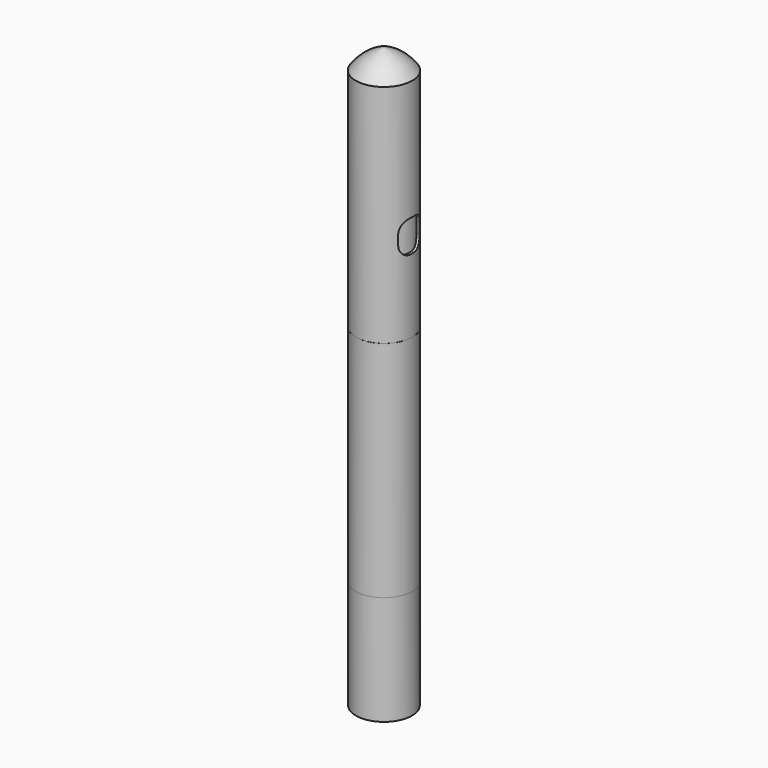
from build123d import *

# Parameters (mm, degrees)
F2_T     = -1
F4_DEPTH = 21.9
F6_E12_W = 45.703087002
F6_E12_H = 50
F7_DEPTH = 0.01


with BuildPart() as f1:
    # F0 (on Front) → F1 (revolve)
    with BuildSketch(Plane.XZ):
        with BuildLine():
            Line((-10.5, -33.0094280231), (0, -33.0094280231))
            Line((0, -33.0094280231), (0, 176.4999798387))
            Line((0, 176.4999798387), (0, 183.9905719769))
            ThreePointArc((0, 183.9905719769), (-5.9594664964, 181.1784924991), (-10.6, 176.4999798387))
            Line((-10.6, 176.4999798387), (-10.6, 7.9905719769))
            Line((-10.6, 7.9905719769), (-10.5, 7.9905719769))
            Line((-10.5, 7.9905719769), (-10.5, -33.0094280231))
        make_face()
    revolve(axis=Axis((0, 0, 180.2452759078), (0, 0, 1)))

    # F2
    f2_openings = [f1.faces().sort_by_distance(p)[0] for p in [
        (0, 0, -33.009428),
    ]]
    offset(amount=F2_T, openings=f2_openings, kind=Kind.INTERSECTION)

    # F3 (on Right) → F4 (cut)
    with BuildSketch(Plane.YZ):
        with BuildLine():
            ThreePointArc((5, 127.4999798387), (3.8284271247, 130.3284069635), (1, 131.4999798387))
            Line((1, 131.4999798387), (-1, 131.4999798387))
            ThreePointArc((-1, 131.4999798387), (-3.8284271247, 130.3284069635), (-5, 127.4999798387))
            Line((-5, 127.4999798387), (-5, 123.4999798387))
            ThreePointArc((-5, 123.4999798387), (-3.8284271247, 120.671552714), (-1, 119.4999798387))
            Line((-1, 119.4999798387), (1, 119.4999798387))
            ThreePointArc((1, 119.4999798387), (3.8284271247, 120.671552714), (5, 123.4999798387))
            Line((5, 123.4999798387), (5, 127.4999798387))
        make_face()
    extrude(amount=F4_DEPTH, mode=Mode.SUBTRACT)

    # F6_E12 (on explicit) → F7 (cut)
    with BuildSketch(Plane(origin=(-25, 19.7467152029, 91.902948916), x_dir=(0, -1, 0), z_dir=(0, 0, 1))):
        with Locations((22.851543501, 25)):
            Rectangle(F6_E12_W, F6_E12_H)
    extrude(amount=-F7_DEPTH, mode=Mode.SUBTRACT)


solid = f1.part
